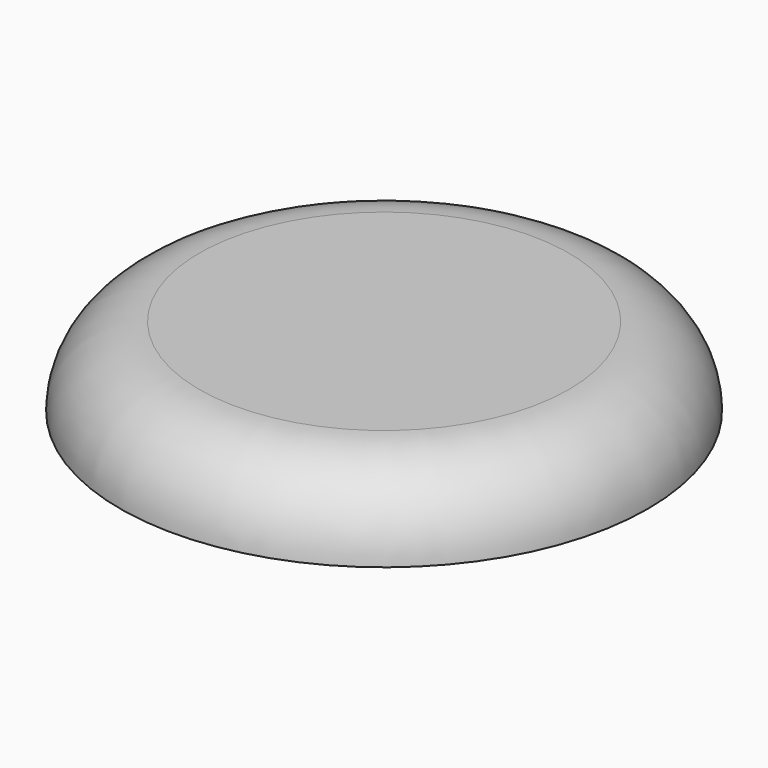
from build123d import *

# Parameters (mm, degrees)
F0_R     = 25.4
F1_DEPTH = 7.62
F2_R     = 7.61999


# Not quite as in the source:
# - a fillet or chamfer is up to 0.001 mm smaller than in the source, because OpenCascade refuses the exact size


with BuildPart() as f1:
    # F0 (on Top) → F1 (new body)
    with BuildSketch(Plane.XY):
        Circle(F0_R)
    extrude(amount=F1_DEPTH)

    # F2 (radius 7.62 in the source; OpenCascade refuses exactly that, so slightly less here)
    f2_edges = [f1.edges().sort_by_distance(p)[0] for p in [
        (-25.4, 0, 7.62),
    ]]
    fillet(f2_edges, radius=F2_R)


solid = f1.part
